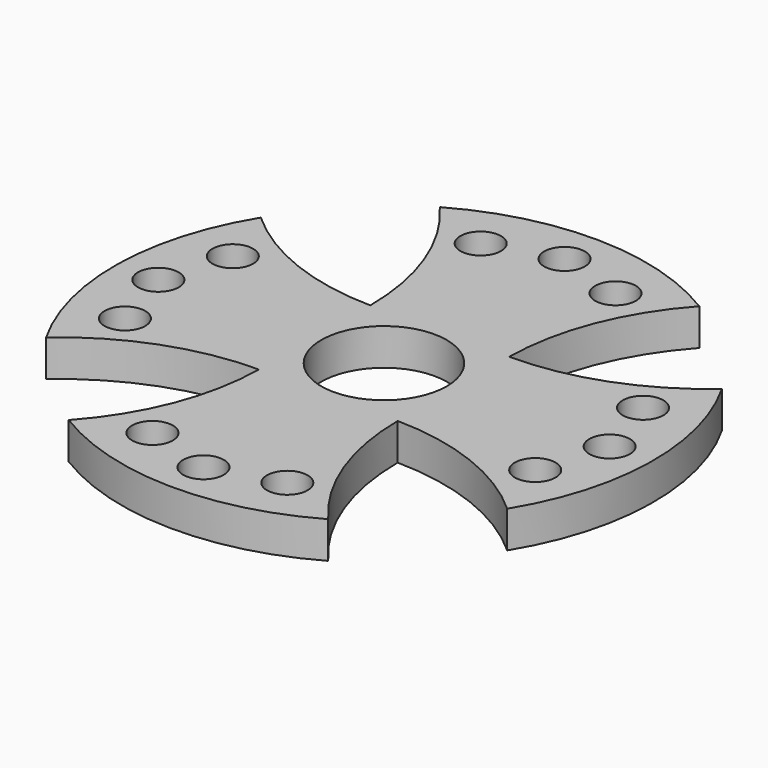
from build123d import *

# Parameters (mm, degrees)
F0_R     = 3.6
F0_R_2   = 11.1
F1_DEPTH = 6.5


with BuildPart() as f1:
    # F0 (on Top) → F1 (new body)
    with BuildSketch(Plane.XY):
        with BuildLine():
            ThreePointArc((12.7551052803, 5.7712467707), (13.2775282625, 2.8640474895), (14, 0))
            ThreePointArc((14, 0), (13.6852379213, 2.951993062), (12.7551052803, 5.7712467707))
        make_face()
        with BuildLine():
            ThreePointArc((12.7551052803, 5.7712467707), (13.6852379213, 2.951993062), (14, 0))
            ThreePointArc((14, 0), (13.6843771554, -2.9559806947), (12.7517397332, -5.7786792415))
            ThreePointArc((12.7517397332, -5.7786792415), (12.3951684194, -9.0411992807), (12.2812401035, -12.3211688608))
            ThreePointArc((12.2812401035, -12.3211688608), (27.4116387343, -15.2593204889), (40.5084826052, -23.3854744583))
            ThreePointArc((40.5084826052, -23.3854744583), (47.2547330266, -0.2211970993), (41.2789992988, 23.1537092477))
            ThreePointArc((41.2789992988, 23.1537092477), (27.7803945414, 15.1065071257), (12.3211688608, 12.2812401035))
            ThreePointArc((12.3211688608, 12.2812401035), (12.4134187433, 9.0179300915), (12.7551052803, 5.7712467707))
        make_face()
        with Locations((36.3028572677, -11.9313535626)):
            Circle(F0_R, mode=Mode.SUBTRACT)
        with Locations((39.9324558712, 0)):
            Circle(F0_R, mode=Mode.SUBTRACT)
        with Locations((36.3028572677, 11.9313535626)):
            Circle(F0_R, mode=Mode.SUBTRACT)
        with BuildLine():
            ThreePointArc((12.7517397332, -5.7786792415), (13.2793138092, -2.8684824171), (14, 0))
            ThreePointArc((14, 0), (13.2775282625, 2.8640474895), (12.7551052803, 5.7712467707))
            ThreePointArc((12.7551052803, 5.7712467707), (9.9023791422, 9.8966098905), (5.7786792415, 12.7517397332))
            ThreePointArc((5.7786792415, 12.7517397332), (2.8684824171, 13.2793138092), (0, 14))
            ThreePointArc((0, 14), (-2.8640474895, 13.2775282625), (-5.7712467707, 12.7551052803))
            ThreePointArc((-5.7712467707, 12.7551052803), (-9.8966098905, 9.9023791422), (-12.7517397332, 5.7786792415))
            ThreePointArc((-12.7517397332, 5.7786792415), (-13.2793138092, 2.8684824171), (-14, 0))
            ThreePointArc((-14, 0), (-13.2775282625, -2.8640474895), (-12.7551052803, -5.7712467707))
            ThreePointArc((-12.7551052803, -5.7712467707), (-9.9023791422, -9.8966098905), (-5.7786792415, -12.7517397332))
            ThreePointArc((-5.7786792415, -12.7517397332), (-2.8684824171, -13.2793138092), (0, -14))
            ThreePointArc((0, -14), (2.8640474895, -13.2775282625), (5.7712467707, -12.7551052803))
            ThreePointArc((5.7712467707, -12.7551052803), (9.8966098905, -9.9023791422), (12.7517397332, -5.7786792415))
        make_face()
        Circle(F0_R_2, mode=Mode.SUBTRACT)
        with BuildLine():
            ThreePointArc((12.7517397332, -5.7786792415), (13.6843771554, -2.9559806947), (14, 0))
            ThreePointArc((14, 0), (13.2793138092, -2.8684824171), (12.7517397332, -5.7786792415))
        make_face()
        with BuildLine():
            ThreePointArc((5.7786792415, 12.7517397332), (9.9023791422, 9.8966098905), (12.7551052803, 5.7712467707))
            ThreePointArc((12.7551052803, 5.7712467707), (12.4134187433, 9.0179300915), (12.3211688608, 12.2812401035))
            ThreePointArc((12.3211688608, 12.2812401035), (9.0411992807, 12.3951684194), (5.7786792415, 12.7517397332))
        make_face()
        with BuildLine():
            ThreePointArc((12.2812401035, -12.3211688608), (12.3951684194, -9.0411992807), (12.7517397332, -5.7786792415))
            ThreePointArc((12.7517397332, -5.7786792415), (9.8966098905, -9.9023791422), (5.7712467707, -12.7551052803))
            ThreePointArc((5.7712467707, -12.7551052803), (9.0179300915, -12.4134187433), (12.2812401035, -12.3211688608))
        make_face()
        with BuildLine():
            ThreePointArc((0, 14), (2.8684824171, 13.2793138092), (5.7786792415, 12.7517397332))
            ThreePointArc((5.7786792415, 12.7517397332), (2.9559806947, 13.6843771554), (0, 14))
        make_face()
        with BuildLine():
            ThreePointArc((0, 14), (2.9559806947, 13.6843771554), (5.7786792415, 12.7517397332))
            ThreePointArc((5.7786792415, 12.7517397332), (9.0411992807, 12.3951684194), (12.3211688608, 12.2812401035))
            ThreePointArc((12.3211688608, 12.2812401035), (15.2593204889, 27.4116387343), (23.3854744583, 40.5084826052))
            ThreePointArc((23.3854744583, 40.5084826052), (0.2211970993, 47.2547330266), (-23.1537092477, 41.2789992988))
            ThreePointArc((-23.1537092477, 41.2789992988), (-15.1065071257, 27.7803945414), (-12.2812401035, 12.3211688608))
            ThreePointArc((-12.2812401035, 12.3211688608), (-9.0179300915, 12.4134187433), (-5.7712467707, 12.7551052803))
            ThreePointArc((-5.7712467707, 12.7551052803), (-2.951993062, 13.6852379213), (0, 14))
        make_face()
        with Locations((-11.9313535626, 36.3028572677)):
            Circle(F0_R, mode=Mode.SUBTRACT)
        with Locations((0, 39.9324558712)):
            Circle(F0_R, mode=Mode.SUBTRACT)
        with Locations((11.9313535626, 36.3028572677)):
            Circle(F0_R, mode=Mode.SUBTRACT)
        with BuildLine():
            ThreePointArc((12.2812401035, -12.3211688608), (9.0179300915, -12.4134187433), (5.7712467707, -12.7551052803))
            ThreePointArc((5.7712467707, -12.7551052803), (2.951993062, -13.6852379213), (0, -14))
            ThreePointArc((0, -14), (-2.9559806947, -13.6843771554), (-5.7786792415, -12.7517397332))
            ThreePointArc((-5.7786792415, -12.7517397332), (-9.0411992807, -12.3951684194), (-12.3211688608, -12.2812401035))
            ThreePointArc((-12.3211688608, -12.2812401035), (-15.2593204889, -27.4116387343), (-23.3854744583, -40.5084826052))
            ThreePointArc((-23.3854744583, -40.5084826052), (-0.2211970993, -47.2547330266), (23.1537092477, -41.2789992988))
            ThreePointArc((23.1537092477, -41.2789992988), (15.1065071257, -27.7803945414), (12.2812401035, -12.3211688608))
        make_face()
        with Locations((-11.9313535626, -36.3028572677)):
            Circle(F0_R, mode=Mode.SUBTRACT)
        with Locations((0, -39.9324558712)):
            Circle(F0_R, mode=Mode.SUBTRACT)
        with Locations((11.9313535626, -36.3028572677)):
            Circle(F0_R, mode=Mode.SUBTRACT)
        with BuildLine():
            ThreePointArc((0, -14), (2.951993062, -13.6852379213), (5.7712467707, -12.7551052803))
            ThreePointArc((5.7712467707, -12.7551052803), (2.8640474895, -13.2775282625), (0, -14))
        make_face()
        with BuildLine():
            ThreePointArc((-5.7712467707, 12.7551052803), (-2.8640474895, 13.2775282625), (0, 14))
            ThreePointArc((0, 14), (-2.951993062, 13.6852379213), (-5.7712467707, 12.7551052803))
        make_face()
        with BuildLine():
            ThreePointArc((-5.7786792415, -12.7517397332), (-2.9559806947, -13.6843771554), (0, -14))
            ThreePointArc((0, -14), (-2.8684824171, -13.2793138092), (-5.7786792415, -12.7517397332))
        make_face()
        with BuildLine():
            ThreePointArc((-12.7517397332, 5.7786792415), (-9.8966098905, 9.9023791422), (-5.7712467707, 12.7551052803))
            ThreePointArc((-5.7712467707, 12.7551052803), (-9.0179300915, 12.4134187433), (-12.2812401035, 12.3211688608))
            ThreePointArc((-12.2812401035, 12.3211688608), (-12.3951684194, 9.0411992807), (-12.7517397332, 5.7786792415))
        make_face()
        with BuildLine():
            ThreePointArc((-12.3211688608, -12.2812401035), (-9.0411992807, -12.3951684194), (-5.7786792415, -12.7517397332))
            ThreePointArc((-5.7786792415, -12.7517397332), (-9.9023791422, -9.8966098905), (-12.7551052803, -5.7712467707))
            ThreePointArc((-12.7551052803, -5.7712467707), (-12.4134187433, -9.0179300915), (-12.3211688608, -12.2812401035))
        make_face()
        with BuildLine():
            ThreePointArc((-14, 0), (-13.2793138092, 2.8684824171), (-12.7517397332, 5.7786792415))
            ThreePointArc((-12.7517397332, 5.7786792415), (-13.6843771554, 2.9559806947), (-14, 0))
        make_face()
        with BuildLine():
            ThreePointArc((-14, 0), (-13.6843771554, 2.9559806947), (-12.7517397332, 5.7786792415))
            ThreePointArc((-12.7517397332, 5.7786792415), (-12.3951684194, 9.0411992807), (-12.2812401035, 12.3211688608))
            ThreePointArc((-12.2812401035, 12.3211688608), (-27.4116387343, 15.2593204889), (-40.5084826052, 23.3854744583))
            ThreePointArc((-40.5084826052, 23.3854744583), (-47.2547330266, 0.2211970993), (-41.2789992988, -23.1537092477))
            ThreePointArc((-41.2789992988, -23.1537092477), (-27.7803945414, -15.1065071257), (-12.3211688608, -12.2812401035))
            ThreePointArc((-12.3211688608, -12.2812401035), (-12.4134187433, -9.0179300915), (-12.7551052803, -5.7712467707))
            ThreePointArc((-12.7551052803, -5.7712467707), (-13.6852379213, -2.951993062), (-14, 0))
        make_face()
        with Locations((-36.3028572677, -11.9313535626)):
            Circle(F0_R, mode=Mode.SUBTRACT)
        with Locations((-39.9324558712, 0)):
            Circle(F0_R, mode=Mode.SUBTRACT)
        with Locations((-36.3028572677, 11.9313535626)):
            Circle(F0_R, mode=Mode.SUBTRACT)
        with BuildLine():
            ThreePointArc((-14, 0), (-13.6852379213, -2.951993062), (-12.7551052803, -5.7712467707))
            ThreePointArc((-12.7551052803, -5.7712467707), (-13.2775282625, -2.8640474895), (-14, 0))
        make_face()
    extrude(amount=F1_DEPTH)


solid = f1.part
